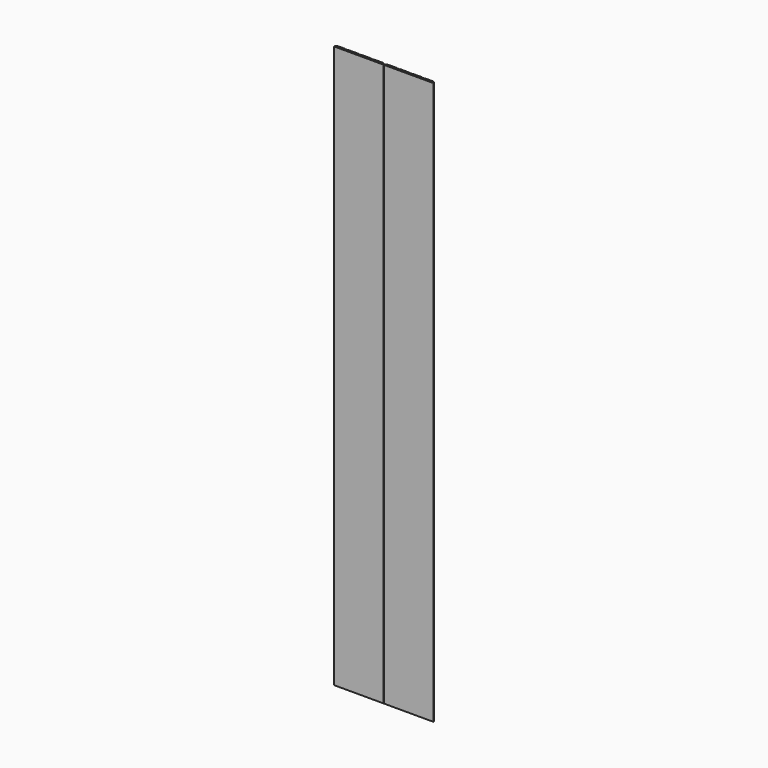
from build123d import *

# Parameters (mm, degrees)
F1_DEPTH    = 704
F3_DEPTH    = 704.001
F4_T1_DEPTH = 713.6824583655
F5_T1_DEPTH = 705.0048304175
F8_W        = 165.4744656086
F8_H        = 350.9649447352
F9_DEPTH    = 1.501


# Not quite as in the source:
# - a fillet or chamfer that OpenCascade refuses, or shapes differently, is made with other operations: its cross-section is extruded or revolved along the edge and cut away or added


with BuildPart() as f1:
    # F0 (on Top) → F1 (new body)
    with BuildSketch(Plane.XY):
        with BuildLine():
            Line((0, 7.5), (0, 0))
            Line((0, 0), (1.5, 0))
            Line((1.5, 0), (1.5, 33.5))
            ThreePointArc((1.5, 33.5), (1.5761204675, 33.8826834324), (1.7928932188, 34.2071067812))
            ThreePointArc((1.7928932188, 34.2071067812), (2.1173165676, 34.4238795325), (2.5, 34.5))
            Line((2.5, 34.5), (36, 34.5))
            Line((36, 34.5), (36, 36))
            Line((36, 36), (28.5, 36))
            Line((28.5, 36), (28.5, 35.75))
            Line((28.5, 35.75), (26.5, 35.75))
            Line((26.5, 35.75), (26.5, 36))
            Line((26.5, 36), (20, 36))
            Line((20, 36), (20, 35.75))
            Line((20, 35.75), (18, 35.75))
            Line((18, 35.75), (18, 36))
            Line((18, 36), (11.5, 36))
            Line((11.5, 36), (11.5, 35.75))
            Line((11.5, 35.75), (9.5, 35.75))
            Line((9.5, 35.75), (9.5, 36))
            Line((9.5, 36), (2, 36))
            ThreePointArc((2, 36), (1.2346331353, 35.847759065), (0.5857864376, 35.4142135624))
            ThreePointArc((0.5857864376, 35.4142135624), (0.152240935, 34.7653668647), (0, 34))
            Line((0, 34), (0, 26.5))
            Line((0, 26.5), (0.25, 26.5))
            Line((0.25, 26.5), (0.25, 24.5))
            Line((0.25, 24.5), (0, 24.5))
            Line((0, 24.5), (0, 18))
            Line((0, 18), (0.25, 18))
            Line((0.25, 18), (0.25, 16))
            Line((0.25, 16), (0, 16))
            Line((0, 16), (0, 9.5))
            Line((0, 9.5), (0.25, 9.5))
            Line((0.25, 9.5), (0.25, 7.5))
            Line((0.25, 7.5), (0, 7.5))
        make_face()
    extrude(amount=F1_DEPTH)

    # F2 (on face) → F3 (cut, through all)
    with BuildSketch(Plane.XY.offset(704)):
        with BuildLine():
            Line((2, 36), (3, 36))
            Line((3, 36), (3, 37.0590753547))
            Line((3, 37.0590753547), (0, 37.0590753547))
            Line((0, 37.0590753547), (0, 34))
            ThreePointArc((0, 34), (0.5857864376, 35.4142135624), (2, 36))
        make_face()
        with BuildLine():
            Line((1.5, 33.5), (1.5, 0))
            Line((1.5, 0), (3, 0))
            Line((3, 0), (3, 34.5))
            Line((3, 34.5), (2.5, 34.5))
            ThreePointArc((2.5, 34.5), (1.7928932188, 34.2071067812), (1.5, 33.5))
        make_face()
        with BuildLine():
            Line((0, 7.5), (0, 0))
            Line((0, 0), (1.5, 0))
            Line((1.5, 0), (1.5, 33.5))
            ThreePointArc((1.5, 33.5), (1.7928932188, 34.2071067812), (2.5, 34.5))
            Line((2.5, 34.5), (3, 34.5))
            Line((3, 34.5), (3, 36))
            Line((3, 36), (2, 36))
            ThreePointArc((2, 36), (0.5857864376, 35.4142135624), (0, 34))
            Line((0, 34), (0, 26.5))
            Line((0, 26.5), (0.25, 26.5))
            Line((0.25, 26.5), (0.25, 24.5))
            Line((0.25, 24.5), (0, 24.5))
            Line((0, 24.5), (0, 18))
            Line((0, 18), (0.25, 18))
            Line((0.25, 18), (0.25, 16))
            Line((0.25, 16), (0, 16))
            Line((0, 16), (0, 9.5))
            Line((0, 9.5), (0.25, 9.5))
            Line((0.25, 9.5), (0.25, 7.5))
            Line((0.25, 7.5), (0, 7.5))
        make_face()
    extrude(amount=-F3_DEPTH, mode=Mode.SUBTRACT)

    # F4: fillet of radius 2 on 2 edges, made by hand

    # F4_s2 → F4_t1 (cut)
    with BuildSketch(Plane.XY.offset(-4.8412291828)):
        with BuildLine():
            ThreePointArc((3, 34.5), (3.7117468017, 35.5811388301), (4.9364916731, 36))
            Line((4.9364916731, 36), (3, 36))
            Line((3, 36), (3, 34.5))
        make_face()
        with BuildLine():
            ThreePointArc((34.0635083269, 36), (35.2882531983, 35.5811388301), (36, 34.5))
            Line((36, 34.5), (36, 36))
            Line((36, 36), (34.0635083269, 36))
        make_face()
    extrude(amount=F4_T1_DEPTH, mode=Mode.SUBTRACT)

    # F5: fillet of radius 0.2 on 6 edges, made by hand

    # F5_s2 → F5_t1 (cut)
    with BuildSketch(Plane.XY.offset(-0.5024152088)):
        with BuildLine():
            ThreePointArc((17.7990343146, 36.0004), (17.9414213562, 35.9414213562), (18.0004, 35.7990343146))
            Line((18.0004, 35.7990343146), (18.0205365685, 35.7990343146))
            ThreePointArc((18.0205365685, 35.7990343146), (18.0201365685, 35.8995171573), (18.0201365685, 36))
            Line((18.0201365685, 36), (18, 36.0201365685))
            ThreePointArc((18, 36.0201365685), (17.8995171573, 36.0201365685), (17.7990343146, 36.0205365685))
            Line((17.7990343146, 36.0205365685), (17.7990343146, 36.0004))
        make_face()
        with BuildLine():
            ThreePointArc((19.9996, 35.7990343146), (20.0585786438, 35.9414213562), (20.2009656854, 36.0004))
            Line((20.2009656854, 36.0004), (20.2009656854, 36.0205365685))
            ThreePointArc((20.2009656854, 36.0205365685), (20.1004828427, 36.0201365685), (20, 36.0201365685))
            Line((20, 36.0201365685), (19.9798634315, 36))
            ThreePointArc((19.9798634315, 36), (19.9798634315, 35.8995171573), (19.9794634315, 35.7990343146))
            Line((19.9794634315, 35.7990343146), (19.9996, 35.7990343146))
        make_face()
        with BuildLine():
            ThreePointArc((28.4996, 35.7990343146), (28.5585786438, 35.9414213562), (28.7009656854, 36.0004))
            Line((28.7009656854, 36.0004), (28.7009656854, 36.0205365685))
            ThreePointArc((28.7009656854, 36.0205365685), (28.6004828427, 36.0201365685), (28.5, 36.0201365685))
            Line((28.5, 36.0201365685), (28.4798634315, 36))
            ThreePointArc((28.4798634315, 36), (28.4798634315, 35.8995171573), (28.4794634315, 35.7990343146))
            Line((28.4794634315, 35.7990343146), (28.4996, 35.7990343146))
        make_face()
        with BuildLine():
            ThreePointArc((26.2990343146, 36.0004), (26.4414213562, 35.9414213562), (26.5004, 35.7990343146))
            Line((26.5004, 35.7990343146), (26.5205365685, 35.7990343146))
            ThreePointArc((26.5205365685, 35.7990343146), (26.5201365685, 35.8995171573), (26.5201365685, 36))
            Line((26.5201365685, 36), (26.5, 36.0201365685))
            ThreePointArc((26.5, 36.0201365685), (26.3995171573, 36.0201365685), (26.2990343146, 36.0205365685))
            Line((26.2990343146, 36.0205365685), (26.2990343146, 36.0004))
        make_face()
        with BuildLine():
            ThreePointArc((9.2990343146, 36.0004), (9.4414213562, 35.9414213562), (9.5004, 35.7990343146))
            Line((9.5004, 35.7990343146), (9.5205365685, 35.7990343146))
            ThreePointArc((9.5205365685, 35.7990343146), (9.5201365685, 35.8995171573), (9.5201365685, 36))
            Line((9.5201365685, 36), (9.5, 36.0201365685))
            ThreePointArc((9.5, 36.0201365685), (9.3995171573, 36.0201365685), (9.2990343146, 36.0205365685))
            Line((9.2990343146, 36.0205365685), (9.2990343146, 36.0004))
        make_face()
        with BuildLine():
            ThreePointArc((11.4996, 35.7990343146), (11.5585786438, 35.9414213562), (11.7009656854, 36.0004))
            Line((11.7009656854, 36.0004), (11.7009656854, 36.0205365685))
            ThreePointArc((11.7009656854, 36.0205365685), (11.6004828427, 36.0201365685), (11.5, 36.0201365685))
            Line((11.5, 36.0201365685), (11.4798634315, 36))
            ThreePointArc((11.4798634315, 36), (11.4798634315, 35.8995171573), (11.4794634315, 35.7990343146))
            Line((11.4794634315, 35.7990343146), (11.4996, 35.7990343146))
        make_face()
    extrude(amount=F5_T1_DEPTH, mode=Mode.SUBTRACT)


with BuildPart() as f7_1:
    # F7: instance of F1
    add(f1.part.mirror(Plane.YZ.offset(36.1)))


with BuildPart() as f9_tool:
    # F8 (on face) → F9 (new body, through all)
    with BuildSketch(Plane.XZ.offset(-34.5)):
        with Locations((85.7372328043, 154.5175276324)):
            Rectangle(F8_W, F8_H)
    extrude(amount=-F9_DEPTH)


with BuildPart() as f1_1:
    add(f1.part)

    # F9: cut by f9_tool
    add(f9_tool.part, mode=Mode.SUBTRACT)


with BuildPart() as f7_1_1:
    add(f7_1.part)

    # F9: cut by f9_tool
    add(f9_tool.part, mode=Mode.SUBTRACT)


solid = Compound([f1_1.part, f7_1_1.part])
